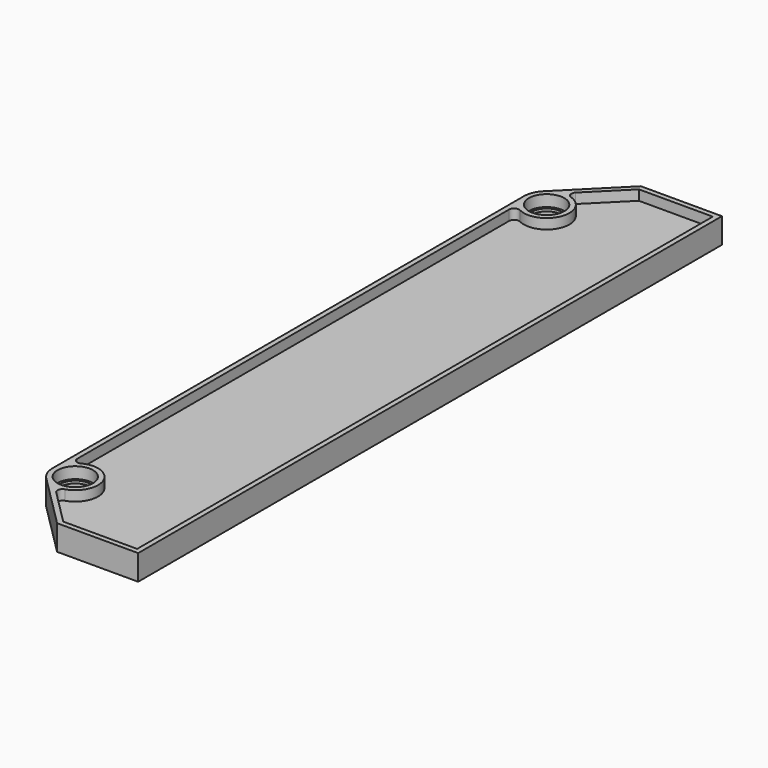
from build123d import *

# Parameters (mm, degrees)
F0_R      = 9.525
F1_DEPTH  = 15.8115
F2_R      = 11.1125
F3_DEPTH  = 7.112
F4_R      = 11.1125
F5_DEPTH  = 7.112
F6_T      = 3.175
F7_R      = 3.175
F8_DEPTH  = 3.175
F10_R     = 11.1125
F11_DEPTH = 1.5875


# Not quite as in the source:
# - a shell that OpenCascade refuses in one call is made with other operations: the cavity is built on its own and cut out


with BuildPart() as f1:
    # F0 (on Top) → F1 (new body)
    with BuildSketch(Plane.XY):
        with BuildLine():
            Line((-14.2875, 369.1638474552), (-14.2875, 0))
            ThreePointArc((-14.2875, 0), (-13.1999288208, -5.4675895399), (-10.1027881362, -10.1027881362))
            Line((-10.1027881362, -10.1027881362), (23.8125, -44.0180762724))
            Line((23.8125, -44.0180762724), (74.6125, -44.0180762724))
            Line((74.6125, -44.0180762724), (74.6125, 413.1819237276))
            Line((74.6125, 413.1819237276), (23.8125, 413.1819237276))
            Line((23.8125, 413.1819237276), (-10.1027881362, 379.2666355914))
            ThreePointArc((-10.1027881362, 379.2666355914), (-13.1999288208, 374.6314369951), (-14.2875, 369.1638474552))
        make_face()
        Circle(F0_R, mode=Mode.SUBTRACT)
        with Locations((0, 369.1638474552)):
            Circle(F0_R, mode=Mode.SUBTRACT)
    extrude(amount=F1_DEPTH)

    # F2 (on face) → F3 (cut)
    with BuildSketch(Plane.XY.offset(15.8115)):
        with Locations((0, 369.1638474552)):
            Circle(F2_R)
        Circle(F2_R)
    extrude(amount=-F3_DEPTH, mode=Mode.SUBTRACT)

    # F4 (on face) → F5 (cut)
    with BuildSketch(Plane(origin=(0, 0, 0), x_dir=(1, 0, 0), z_dir=(0, 0, -1))):
        Circle(F4_R)
        with Locations((0, -369.1638474552)):
            Circle(F4_R)
    extrude(amount=-F5_DEPTH, mode=Mode.SUBTRACT)

    # F6: shell of thickness 3.175, made by hand


with BuildPart() as f6_core1:
    # F6_t2: copy of F1
    add(f1.part)

    # the walls: a layer under each face that stays
    f6_faces = [f6_core1.faces().sort_by_distance(p)[0] for p in [
        (-13.1999288208, 374.6314369951, 7.90575),
        (6.8548559319, 396.2242796595, 7.90575),
        (-14.2875, 184.5819237276, 7.90575),
        (30.1625, 184.5819237276, 15.8115),
        (49.2125, 413.1819237276, 7.90575),
        (-13.1999288208, -5.4675895399, 7.90575),
        (74.6125, 184.5819237276, 7.90575),
        (6.8548559319, -27.0604322043, 7.90575),
        (49.2125, -44.0180762724, 7.90575),
        (-11.1125, 0, 3.556),
        (-11.1125, 369.1638474552, 3.556),
        (-11.1125, 0, 12.2555),
        (-11.1125, 369.1638474552, 12.2555),
        (-7.4083333333, 7.4083333333, 7.112),
        (-7.4083333333, 376.5721807885, 7.112),
        (-7.4083333333, -7.4083333333, 8.6995),
        (-7.4083333333, 361.7555141219, 8.6995),
        (-9.525, 0, 7.90575),
        (-9.525, 369.1638474552, 7.90575),
    ]]
    thicken(f6_faces, amount=-F6_T, mode=Mode.SUBTRACT)

    # F6_s3 → F6_t4 (revolve, cut)
    with BuildSketch(Plane.XZ):
        Polygon((11.08075, 7.08025), (14.2875, 7.112), (14.2875, 10.287), (11.1125, 10.287), align=None)
    revolve(axis=Axis((0, 0, 7.112), (0, 0, -1)), mode=Mode.SUBTRACT)

    # F6_s5 → F6_t6 (revolve, cut)
    with BuildSketch(Plane.XZ.offset(-369.1638474552)):
        Polygon((11.08075, 7.08025), (14.2875, 7.112), (14.2875, 10.287), (11.1125, 10.287), align=None)
    revolve(axis=Axis((0, 369.1638474552, 7.112), (0, 0, -1)), mode=Mode.SUBTRACT)

    # F6_s7 → F6_t8 (revolve, cut)
    with BuildSketch(Plane.XZ):
        Polygon((11.08075, 8.73125), (14.2875, 8.6995), (14.2875, 5.5245), (11.1125, 5.5245), align=None)
    revolve(axis=Axis((0, 0, 8.6995), (0, 0, 1)), mode=Mode.SUBTRACT)

    # F6_s9 → F6_t10 (revolve, cut)
    with BuildSketch(Plane.XZ.offset(-369.1638474552)):
        Polygon((11.08075, 8.73125), (14.2875, 8.6995), (14.2875, 5.5245), (11.1125, 5.5245), align=None)
    revolve(axis=Axis((0, 369.1638474552, 8.6995), (0, 0, 1)), mode=Mode.SUBTRACT)


with BuildPart() as f1_1:
    add(f1.part)

    # what is left inside the walls is the cavity
    f6_cavity = [f6_core1.part.solids().sort_by_distance(p)[0] for p in [
        (30.1625, 109.440257, 12.60475),
    ]]
    add(f6_cavity, mode=Mode.SUBTRACT)

    # F7
    f7_edges = [f1_1.edges().sort_by_distance(p)[0] for p in [
        (-1.507724, 383.371572, 6.31825),
        (-11.1125, 360.183591, 6.31825),
        (-11.1125, 8.980256, 6.31825),
        (-1.507724, -14.207724, 6.31825),
    ]]
    fillet(f7_edges, radius=F7_R)

    # F8 (cut, through all): a face of the model
    f8_faces = [f1_1.faces().sort_by_distance(p)[0] for p in [
        (32.2546535053, 184.5819237276, 12.6365),
    ]]
    extrude(f8_faces, amount=-F8_DEPTH, mode=Mode.SUBTRACT)

    # F10 (on offset) → F11 (join, symmetric)
    with BuildSketch(Plane.XY.offset(7.90575)):
        with BuildLine():
            Line((74.6125, -44.0180762724), (74.6125, 413.1819237276))
            Line((74.6125, 413.1819237276), (23.8125, 413.1819237276))
            Line((23.8125, 413.1819237276), (-10.1027881362, 379.2666355914))
            ThreePointArc((-10.1027881362, 379.2666355914), (-13.1999288208, 374.6314369951), (-14.2875, 369.1638474552))
            Line((-14.2875, 369.1638474552), (-14.2875, 0))
            ThreePointArc((-14.2875, 0), (-13.1999288208, -5.4675895399), (-10.1027881362, -10.1027881362))
            Line((-10.1027881362, -10.1027881362), (23.8125, -44.0180762724))
            Line((23.8125, -44.0180762724), (74.6125, -44.0180762724))
        make_face()
        Circle(F10_R, mode=Mode.SUBTRACT)
        with Locations((0, 369.1638474552)):
            Circle(F10_R, mode=Mode.SUBTRACT)
    extrude(amount=F11_DEPTH, both=True)


solid = f1_1.part
